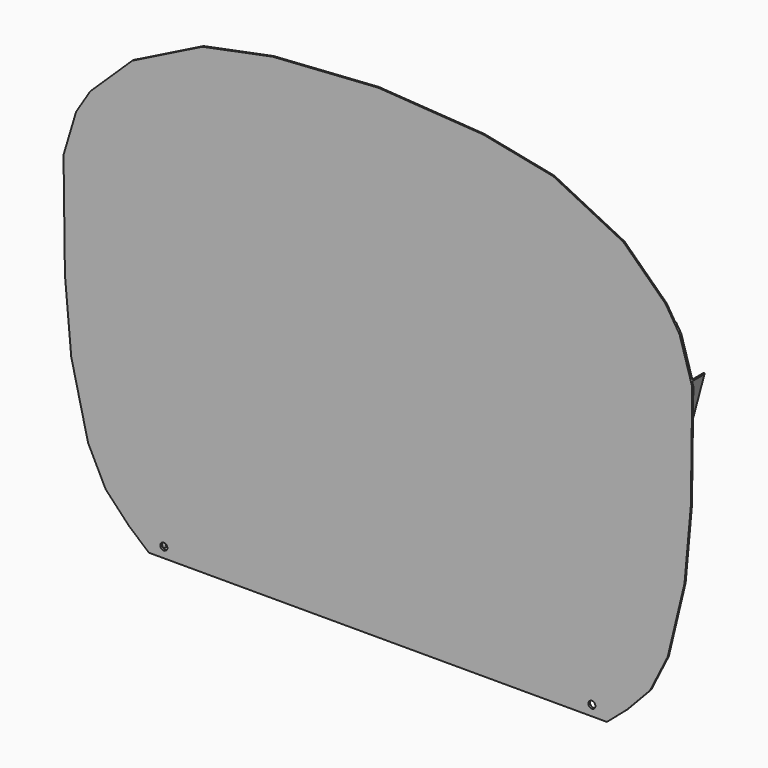
from build123d import *

# Parameters (mm, degrees)
F0_R     = 5
F1_DEPTH = 2
F2_DEPTH = 1
F3_DEPTH = 22
F4_SIZE2 = 0.352644
F4_SIZE  = 1.99999


# Not quite as in the source:
# - a fillet or chamfer is up to 0.001 mm smaller than in the source, because OpenCascade refuses the exact size


with BuildPart() as f1:
    # F0 (on Front) → F1 (new body)
    with BuildSketch(Plane.XZ):
        Polygon((-202.1265400052, 210), (-217.8300492651, 157.6549691337), (-92.7831770837, -310), (-52.4130318677, -310), (-194.6536201768, 221.9566717254), align=None)
        with Locations((-77.1265400052, -295)):
            Circle(F0_R, mode=Mode.SUBTRACT)
        Polygon((-182.1265400052, 242), (-194.6536201768, 221.9566717254), (-52.4130318677, -310), (227.8734599948, -310), (508.1599518573, -310), (650.4005401664, 221.9566717254), (637.8734599948, 242), (577.8734599948, 300), (477.8734599948, 350), (377.8734599948, 370), (227.8734599948, 380), (77.8734599948, 370), (-22.1265400052, 350), (-122.1265400052, 300), align=None)
        Polygon((650.4005401664, 221.9566717254), (508.1599518573, -310), (548.5300970733, -310), (673.5769692547, 157.6549691337), (657.8734599948, 210), align=None)
        with Locations((532.8734599948, -295)):
            Circle(F0_R, mode=Mode.SUBTRACT)
        Polygon((-220.1265400052, 150), (-218.1265400052, 0), (-209.1265400052, -100), (-185.1265400052, -200), (-160.1265400052, -250), (-127.1265400052, -285), (-98.1265400052, -310), (-93.8183090123, -310), (-218.3773603998, 155.8305986848), align=None)
        Polygon((674.1242803894, 155.8305986848), (549.5652290019, -310), (553.8734599948, -310), (582.8734599948, -285), (615.8734599948, -250), (640.8734599948, -200), (664.8734599948, -100), (673.8734599948, 0), (675.8734599948, 150), align=None)
        Polygon((673.5769692547, 157.6549691337), (548.5300970733, -310), (549.5652290019, -310), (674.1242803894, 155.8305986848), align=None)
        Polygon((-217.8300492651, 157.6549691337), (-218.3773603998, 155.8305986848), (-93.8183090123, -310), (-92.7831770837, -310), align=None)
    extrude(amount=F1_DEPTH)

    # F0 (on Front) → F2 (join)
    with BuildSketch(Plane.XZ):
        Polygon((-202.1265400052, 210), (-217.8300492651, 157.6549691337), (-92.7831770837, -310), (-52.4130318677, -310), (-194.6536201768, 221.9566717254), align=None)
        with Locations((-77.1265400052, -295)):
            Circle(F0_R, mode=Mode.SUBTRACT)
        Polygon((650.4005401664, 221.9566717254), (508.1599518573, -310), (548.5300970733, -310), (673.5769692547, 157.6549691337), (657.8734599948, 210), align=None)
        with Locations((532.8734599948, -295)):
            Circle(F0_R, mode=Mode.SUBTRACT)
    extrude(amount=-F2_DEPTH)

    # F0 (on Front) → F3 (join)
    with BuildSketch(Plane.XZ):
        Polygon((673.5769692547, 157.6549691337), (548.5300970733, -310), (549.5652290019, -310), (674.1242803894, 155.8305986848), align=None)
        Polygon((-217.8300492651, 157.6549691337), (-218.3773603998, 155.8305986848), (-93.8183090123, -310), (-92.7831770837, -310), align=None)
    extrude(amount=-F3_DEPTH)

    # F4 (size 2 and 0.3526539614 in the source; OpenCascade refuses exactly that, so slightly less here)
    f4_edges = [f1.edges().sort_by_distance(p)[0] for p in [
        (227.87346, -2, -310),
    ]]
    f4_side = f1.faces().sort_by_distance((227.87346, -0.533198, -310))[0]
    chamfer(f4_edges, length=F4_SIZE, length2=F4_SIZE2, reference=f4_side)


solid = f1.part
